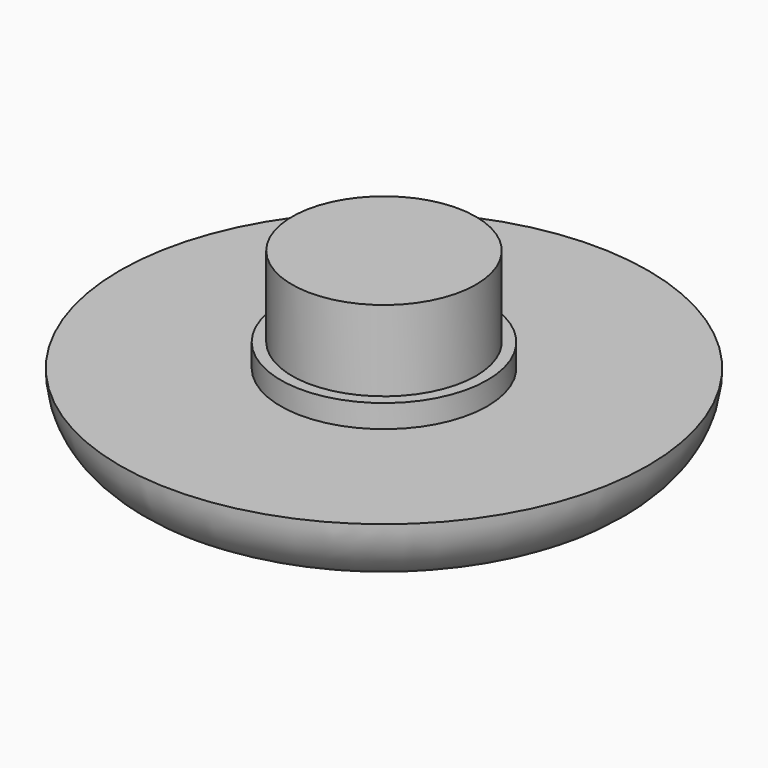
from build123d import *

# Parameters (mm, degrees)
F0_R     = 4.5
F0_R_2   = 4.005
F1_DEPTH = 1
F2_DEPTH = 4.5
F0_R_3   = 11.5
F3_DEPTH = 3
F4_DEPTH = 3
F5_R     = 2.99999


# Not quite as in the source:
# - a fillet or chamfer is up to 0.001 mm smaller than in the source, because OpenCascade refuses the exact size


with BuildPart() as f1:
    # F0 (on Top) → F1 (new body)
    with BuildSketch(Plane.XY):
        Circle(F0_R)
        Circle(F0_R_2, mode=Mode.SUBTRACT)
    extrude(amount=F1_DEPTH)

    # F0 (on Top) → F2 (join)
    with BuildSketch(Plane.XY):
        Circle(F0_R_2)
    extrude(amount=F2_DEPTH)

    # F0 (on Top) → F3 (join)
    with BuildSketch(Plane.XY):
        Circle(F0_R_3)
        Circle(F0_R, mode=Mode.SUBTRACT)
    extrude(amount=-F3_DEPTH)

    # F0 (on Top) → F4 (join)
    with BuildSketch(Plane.XY):
        Circle(F0_R)
        Circle(F0_R_2, mode=Mode.SUBTRACT)
        Circle(F0_R_2)
    extrude(amount=-F4_DEPTH)

    # F5 (radius 3 in the source; OpenCascade refuses exactly that, so slightly less here)
    f5_edges = [f1.edges().sort_by_distance(p)[0] for p in [
        (-11.5, 0, -3),
    ]]
    fillet(f5_edges, radius=F5_R)


solid = f1.part
